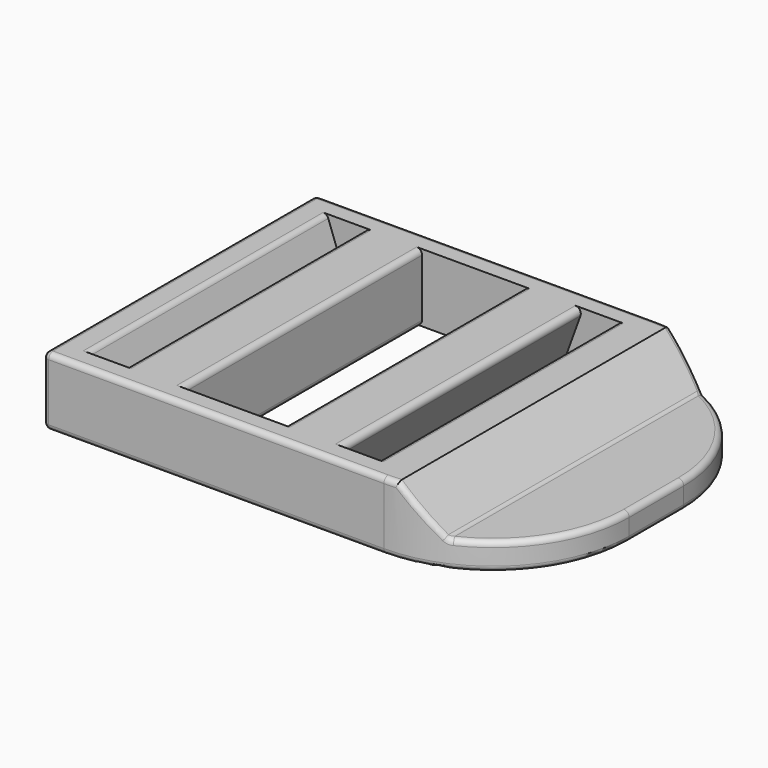
from build123d import *

# Parameters (mm, degrees)
F0_W     = 44.45
F0_H     = 31.75
F1_DEPTH = 6.35
F2_W     = 9.525
F2_H     = 6.35
F3_DEPTH = 13.97
F5_DEPTH = 31.751
F6_R     = 12.7
F7_R     = 0.508


with BuildPart() as f1:
    # F0 (on Top) → F1 (new body)
    with BuildSketch(Plane.XY):
        Rectangle(F0_W, F0_H)
    extrude(amount=F1_DEPTH)

    # F2 (on Front) → F3 (cut, symmetric)
    with BuildSketch(Plane.XZ):
        with Locations((-6.0325, 3.175)):
            Rectangle(F2_W, F2_H)
        Polygon((-17.1641401403, 8.7758279101), (-20.1476642113, 7.6899139551), (-16.8610756315, -1.3399139551), (-13.8775515605, -0.254), align=None)
        Polygon((1.8125515605, -0.254), (4.7960756315, -1.3399139551), (8.0826642113, 7.6899139551), (5.0991401403, 8.7758279101), align=None)
    extrude(amount=F3_DEPTH, both=True, mode=Mode.SUBTRACT)

    # F4 (on face) → F5 (cut, through all)
    with BuildSketch(Plane.XZ.offset(15.875)):
        Polygon((22.225, 6.35), (10.7699754152, 6.35), (14.5799754152, 2.54), (22.225, 2.54), align=None)
    extrude(amount=-F5_DEPTH, mode=Mode.SUBTRACT)

    # F6
    f6_edges = [f1.edges().sort_by_distance(p)[0] for p in [
        (22.225, -15.875, 1.27),
        (22.225, 15.875, 1.27),
    ]]
    fillet(f6_edges, radius=F6_R)

    # F7
    f7_edges = [f1.edges().sort_by_distance(p)[0] for p in [
        (-16.281211, 0, 6.35),
        (-19.659975, 0, 6.35),
        (-17.348764, 0, 0),
        (-10.795, 0, 6.35),
        (-1.27, 0, 6.35),
        (4.216211, 0, 6.35),
        (-13.97, 0, 0),
        (-10.795, 0, 0),
        (-1.27, 0, 0),
        (1.905, 0, 0),
        (5.283764, 0, 0),
        (7.594975, 0, 6.35),
        (14.579975, 0, 2.54),
        (20.143102, -10.142489, 2.54),
        (18.505256, -12.155256, 0),
        (-22.225, 0, 0),
        (-6.35, 15.875, 6.35),
        (-22.225, 0, 6.35),
        (-6.35, -15.875, 6.35),
        (-22.225, -15.875, 3.175),
        (-22.225, 15.875, 3.175),
        (-6.35, 15.875, 0),
        (18.505256, 12.155256, 0),
        (22.225, 0, 0),
        (-6.35, -15.875, 0),
        (10.148239, 15.859698, 6.35),
        (12.713492, 15.468231, 4.406484),
        (20.143102, 10.142489, 2.54),
        (10.148239, -15.859698, 6.35),
        (22.225, 0, 2.54),
        (12.713492, -15.468231, 4.406484),
    ]]
    fillet(f7_edges, radius=F7_R)


solid = f1.part
